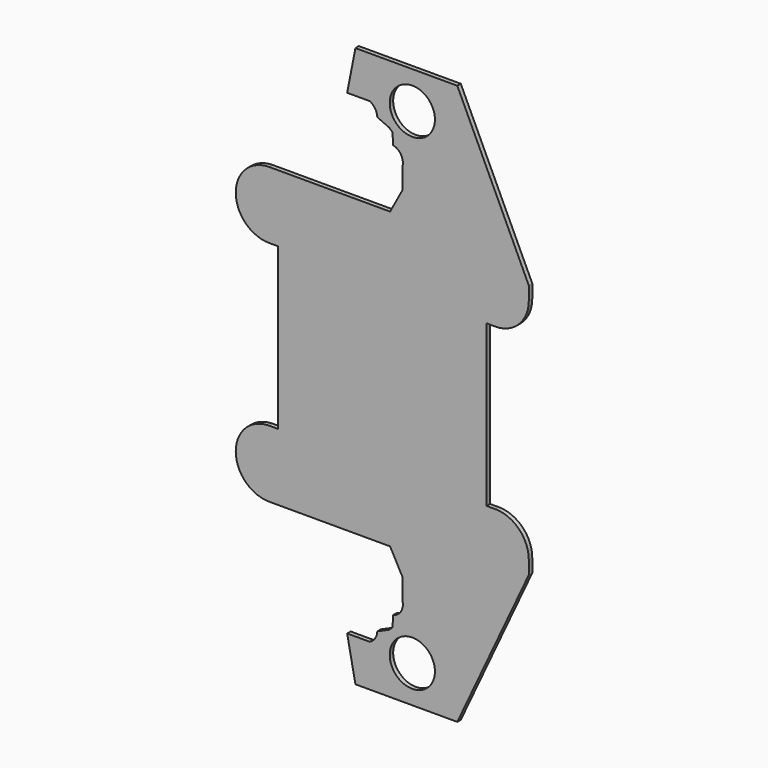
from build123d import *

# Parameters (mm, degrees)
F0_R     = 16.51
F0_W     = 152.420665353
F0_H     = 90.8812
F1_DEPTH = 3.175


# Not quite as in the source:
# - ends of sketch curves that miss each other by under 0.0002 mm in the source are joined
# - a feature names something its author has since deleted; it is built from what else it names


with BuildPart() as f1:
    # F0 (on Front) → F1 (new body)
    with BuildSketch(Plane.XZ):
        with BuildLine():
            Line((65.843271404, -64.4387074201), (72.172606051, -64.494198626))
            ThreePointArc((72.172606051, -64.494198626), (89.5045003647, -57.3150929397), (96.683606051, -39.983198626))
            Line((96.683606051, -39.983198626), (96.683606051, -30.0584486086))
            Line((96.683606051, -30.0584486086), (44.4719158113, 81.3992435336))
            Line((44.4719158113, 81.3992435336), (-29.9480052508, 81.3992435336))
            Line((-29.9480052508, 81.3992435336), (-35.9978974571, 50.6829957967))
            Line((-35.9978974571, 50.6829957967), (-19.4879078689, 50.6714224456))
            ThreePointArc((-19.4879078689, 50.6714224456), (-15.5812211009, 47.1637298884), (-13.9720730804, 42.1660573792))
            Line((-13.9720730804, 42.1660573792), (-5.4024819992, 38.3506346508))
            Line((-5.4024819992, 38.3506346508), (-2.9009456417, 36.1038269705))
            Line((-2.9009456417, 36.1038269705), (-2.3647786124, 27.9011076368))
            ThreePointArc((-2.3647786124, 27.9011076368), (3.4353485173, 23.5426794776), (4.3712937617, 16.3481414632))
            Line((4.3712937617, 16.3481414632), (4.2880776677, 1.0115236557))
            Line((4.2880776677, 1.0115236557), (-4.6405893252, -15.5276898319))
            Line((-4.6405893252, -15.5276898319), (-92.927393949, -15.5276898319))
            ThreePointArc((-92.927393949, -15.5276898319), (-117.3829027431, -39.983198626), (-92.927393949, -64.4387074201))
            Line((-92.927393949, -64.4387074201), (-86.577393949, -64.4387074201))
            Line((-86.577393949, -64.4387074201), (-86.577393949, -77.7312386201))
            Line((-86.577393949, -77.7312386201), (65.843271404, -77.7312386201))
            Line((65.843271404, -77.7312386201), (65.843271404, -64.4387074201))
        make_face()
        with Locations((11.6086210255, 54.3104703533)):
            Circle(F0_R, mode=Mode.SUBTRACT)
        with Locations((-10.3670612725, -123.1718386201)):
            Rectangle(F0_W, F0_H)
        with BuildLine():
            Line((65.843271404, -181.9049698201), (65.843271404, -168.6124386201))
            Line((65.843271404, -168.6124386201), (-86.577393949, -168.6124386201))
            Line((-86.577393949, -168.6124386201), (-86.577393949, -181.9049698201))
            Line((-86.577393949, -181.9049698201), (-92.927393949, -181.9049698201))
            ThreePointArc((-92.927393949, -181.9049698201), (-117.3829027431, -206.3604786142), (-92.927393949, -230.8159874083))
            Line((-92.927393949, -230.8159874083), (-4.6405893252, -230.8159874083))
            Line((-4.6405893252, -230.8159874083), (4.2880776677, -247.355200896))
            Line((4.2880776677, -247.355200896), (4.3712937617, -262.6918187035))
            ThreePointArc((4.3712937617, -262.6918187035), (3.4353485173, -269.8863567179), (-2.3647786124, -274.2447848771))
            Line((-2.3647786124, -274.2447848771), (-2.9009456417, -282.4475042108))
            Line((-2.9009456417, -282.4475042108), (-5.4024819992, -284.6943118911))
            Line((-5.4024819992, -284.6943118911), (-13.9720735102, -288.5097398532))
            ThreePointArc((-13.9720735102, -288.5097398532), (-15.5812211009, -293.5074071287), (-19.487905219, -297.0150996841))
            Line((-19.487905219, -297.0150996841), (-35.9978974571, -297.026673037))
            Line((-35.9978974571, -297.026673037), (-29.9480052508, -327.7429207739))
            Line((-29.9480052508, -327.7429207739), (44.4719158113, -327.7429207739))
            Line((44.4719158113, -327.7429207739), (96.683606051, -216.2852286317))
            Line((96.683606051, -216.2852286317), (96.683606051, -206.3604786142))
            ThreePointArc((96.683606051, -206.3604786142), (89.5045003647, -189.0285843006), (72.172606051, -181.8494786142))
            Line((72.172606051, -181.8494786142), (65.843271404, -181.9049698201))
        make_face()
        with Locations((11.6086210255, -300.6541475936)):
            Circle(F0_R, mode=Mode.SUBTRACT)
    extrude(amount=F1_DEPTH)


solid = f1.part
